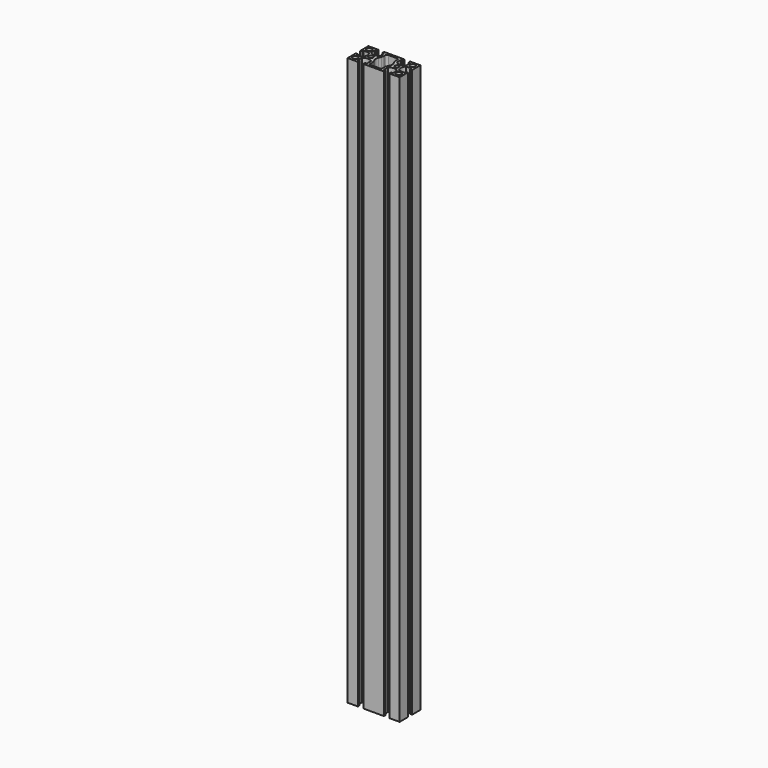
from build123d import *

# Parameters (mm, degrees)
F0_R     = 3
F0_R_2   = 2.5
F1_DEPTH = 655
F2_R     = 2
F3_R     = 7


# Not quite as in the source:
# - a feature names something its author has since deleted; it is built from what else it names


with BuildPart() as f1:
    # F0 (on Top) → F1 (new body)
    with BuildSketch(Plane.XY):
        with BuildLine():
            Line((18.15, -15), (30, -15))
            Line((30, -15), (30, -3.15))
            Line((30, -3.15), (27.5, -3.15))
            Line((27.5, -3.15), (27.5, -5.15))
            Line((27.5, -5.15), (21.5477069044, -5.15))
            ThreePointArc((21.5477069044, -5.15), (19.5, 0), (21.5477069044, 5.15))
            Line((21.5477069044, 5.15), (27.5, 5.15))
            Line((27.5, 5.15), (27.5, 3.15))
            Line((27.5, 3.15), (30, 3.15))
            Line((30, 3.15), (30, 15))
            Line((30, 15), (18.15, 15))
            Line((18.15, 15), (18.15, 12.5))
            Line((18.15, 12.5), (20.15, 12.5))
            Line((20.15, 12.5), (20.15, 6.5477069044))
            ThreePointArc((20.15, 6.5477069044), (15, 4.5), (9.85, 6.5477069044))
            Line((9.85, 6.5477069044), (9.85, 12.5))
            Line((9.85, 12.5), (11.85, 12.5))
            Line((11.85, 12.5), (11.85, 15))
            Line((11.85, 15), (-11.85, 15))
            Line((-11.85, 15), (-11.85, 12.5))
            Line((-11.85, 12.5), (-9.85, 12.5))
            Line((-9.85, 12.5), (-9.85, 6.5477069044))
            ThreePointArc((-9.85, 6.5477069044), (-15, 4.5), (-20.15, 6.5477069044))
            Line((-20.15, 6.5477069044), (-20.15, 12.5))
            Line((-20.15, 12.5), (-18.15, 12.5))
            Line((-18.15, 12.5), (-18.15, 15))
            Line((-18.15, 15), (-30, 15))
            Line((-30, 15), (-30, 3.15))
            Line((-30, 3.15), (-27.5, 3.15))
            Line((-27.5, 3.15), (-27.5, 5.15))
            Line((-27.5, 5.15), (-21.5477069044, 5.15))
            ThreePointArc((-21.5477069044, 5.15), (-19.5, 0), (-21.5477069044, -5.15))
            Line((-21.5477069044, -5.15), (-27.5, -5.15))
            Line((-27.5, -5.15), (-27.5, -3.15))
            Line((-27.5, -3.15), (-30, -3.15))
            Line((-30, -3.15), (-30, -15))
            Line((-30, -15), (-18.15, -15))
            Line((-18.15, -15), (-18.15, -12.5))
            Line((-18.15, -12.5), (-20.15, -12.5))
            Line((-20.15, -12.5), (-20.15, -6.5477069044))
            ThreePointArc((-20.15, -6.5477069044), (-15, -4.5), (-9.85, -6.5477069044))
            Line((-9.85, -6.5477069044), (-9.85, -12.5))
            Line((-9.85, -12.5), (-11.85, -12.5))
            Line((-11.85, -12.5), (-11.85, -15))
            Line((-11.85, -15), (11.85, -15))
            Line((11.85, -15), (11.85, -12.5))
            Line((11.85, -12.5), (9.85, -12.5))
            Line((9.85, -12.5), (9.85, -6.5477069044))
            ThreePointArc((9.85, -6.5477069044), (15, -4.5), (20.15, -6.5477069044))
            Line((20.15, -6.5477069044), (20.15, -12.5))
            Line((20.15, -12.5), (18.15, -12.5))
            Line((18.15, -12.5), (18.15, -15))
        make_face()
        with Locations((-25, -10)):
            Circle(F0_R, mode=Mode.SUBTRACT)
        with Locations((25, -10)):
            Circle(F0_R, mode=Mode.SUBTRACT)
        with Locations((-15, 0)):
            Circle(F0_R_2, mode=Mode.SUBTRACT)
        with Locations((-25, 10)):
            Circle(F0_R, mode=Mode.SUBTRACT)
        Polygon((-7, 7), (-7, 12.5), (0, 12.5), (7, 12.5), (7, 7), (10, 0), (7, -7), (7, -12.5), (0, -12.5), (-7, -12.5), (-7, -7), (-10, 0), align=None, mode=Mode.SUBTRACT)
        with Locations((15, 0)):
            Circle(F0_R_2, mode=Mode.SUBTRACT)
        with Locations((25, 10)):
            Circle(F0_R, mode=Mode.SUBTRACT)
    extrude(amount=F1_DEPTH)

    # F2
    f2_edges = [f1.edges().sort_by_distance(p)[0] for p in [
        (-7, 12.5, 327.5),
        (7, 12.5, 327.5),
    ]]
    fillet(f2_edges, radius=F2_R)

    # F3
    f3_edges = [f1.edges().sort_by_distance(p)[0] for p in [
        (-7, 7, 327.5),
        (-10, 0, 327.5),
        (7, 7, 327.5),
        (10, 0, 327.5),
    ]]
    fillet(f3_edges, radius=F3_R)


solid = f1.part
